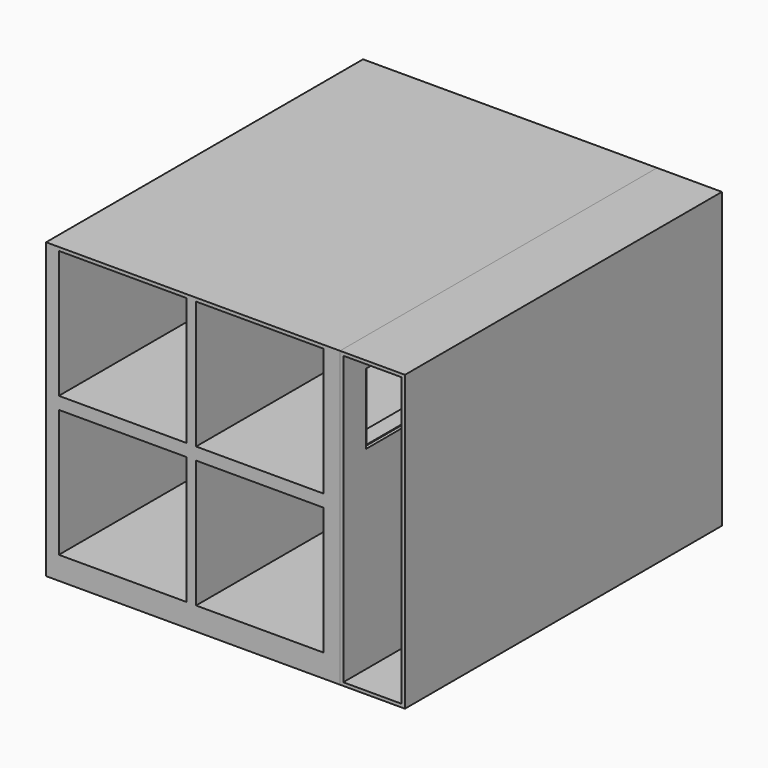
from build123d import *

# Parameters (mm, degrees)
F0_W      = 229.997
F0_H      = 229.997
F1_DEPTH  = 309.99938
F3_DEPTH  = 304.8
F4_W      = 99.822
F4_H      = 99.822
F5_DEPTH  = 304.8
F6_W      = 99.822
F6_H      = 99.822
F7_DEPTH  = 304.8
F8_W      = 99.822
F8_H      = 99.822
F9_DEPTH  = 304.8
F10_DEPTH = 50.8
F11_T     = -2.54
F12_W     = 341.4483144879
F12_H     = 55.3129836917
F13_DEPTH = 32.258
F14_W     = 284.0407041088
F14_H     = 54.226949811
F15_DEPTH = 25.908


with BuildPart() as f1:
    # F0 (on Front) → F1 (new body)
    with BuildSketch(Plane.XZ):
        with Locations((4.1453130543, 40.1437824458)):
            Rectangle(F0_W, F0_H)
    extrude(amount=-F1_DEPTH)

    # F2 (on face) → F3 (cut)
    with BuildSketch(Plane.XZ):
        Polygon((-100.8709869457, 152.4277220995), (-100.8709869457, 127.9133111238), (-100.8709869457, 52.6057220995), (-1.0489869457, 52.6057220995), (-1.0489869457, 152.4277220995), align=None)
    extrude(amount=-F3_DEPTH, mode=Mode.SUBTRACT)

    # F4 (on face) → F5 (cut)
    with BuildSketch(Plane.XZ):
        with Locations((56.4267938881, 102.5167220995)):
            Rectangle(F4_W, F4_H)
    extrude(amount=-F5_DEPTH, mode=Mode.SUBTRACT)

    # F6 (on face) → F7 (cut)
    with BuildSketch(Plane.XZ):
        with Locations((-50.9599869457, -6.994601433)):
            Rectangle(F6_W, F6_H)
    extrude(amount=-F7_DEPTH, mode=Mode.SUBTRACT)

    # F8 (on face) → F9 (cut)
    with BuildSketch(Plane.XZ):
        with Locations((56.4267938881, -6.994601433)):
            Rectangle(F8_W, F8_H)
    extrude(amount=-F9_DEPTH, mode=Mode.SUBTRACT)


with BuildPart() as f10:
    # F10 (new): a face of the model
    f10_faces = [f1.part.faces().sort_by_distance(p)[0] for p in [
        (119.1438130543, 154.99969, 40.1437824458),
    ]]
    extrude(f10_faces, amount=F10_DEPTH)

    # F11
    f11_openings = [f10.faces().sort_by_distance(p)[0] for p in [
        (144.543813, 0, 40.143782),
    ]]
    offset(amount=F11_T, openings=f11_openings)

    # F12 (on face) → F13 (cut)
    with BuildSketch(Plane.YZ.offset(121.6838130543)):
        with Locations((192.8919814527, 107.0070452988)):
            Rectangle(F12_W, F12_H)
    extrude(amount=-F13_DEPTH, mode=Mode.SUBTRACT)


with BuildPart() as f1_1:
    add(f1.part)

    # F14 (on face) → F15 (cut)
    with BuildSketch(Plane.YZ.offset(119.1438130543)):
        with Locations((167.9790279456, 107.128418982)):
            Rectangle(F14_W, F14_H)
    extrude(amount=-F15_DEPTH, mode=Mode.SUBTRACT)


solid = Compound([f10.part, f1_1.part])
